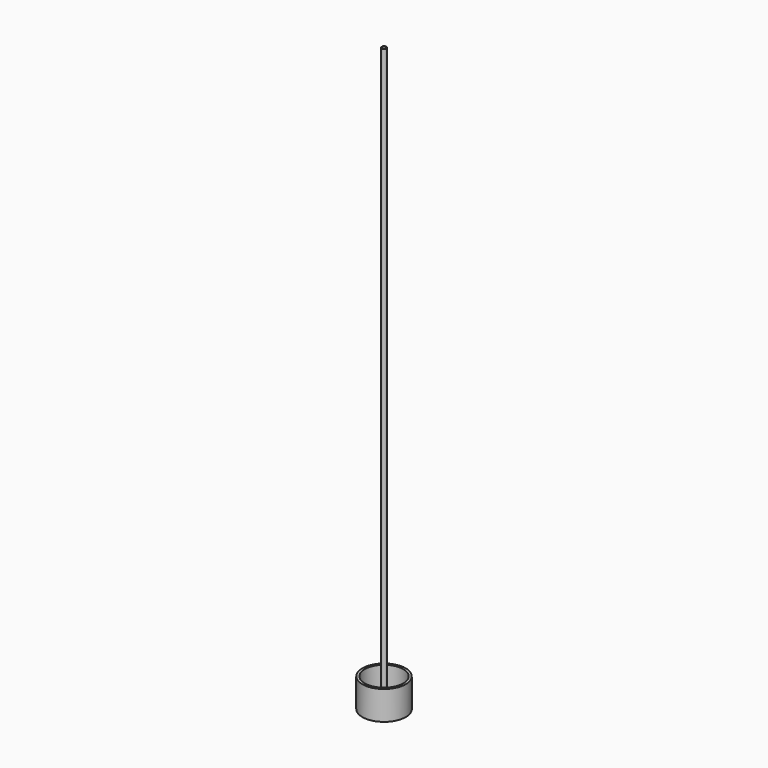
from build123d import *

# Parameters (mm, degrees)
F0_R     = 57.15
F1_DEPTH = 76.2
F2_R     = 50.8
F3_DEPTH = 63.5
F4_R     = 6.35
F4_R_2   = 5.08
F5_DEPTH = 1524


# Not quite as in the source:
# - a fillet or chamfer that OpenCascade refuses, or shapes differently, is made with other operations: its cross-section is extruded or revolved along the edge and cut away or added


with BuildPart() as f1:
    # F0 (on Top) → F1 (new body)
    with BuildSketch(Plane.XY):
        Circle(F0_R)
    extrude(amount=F1_DEPTH)

    # F2 (on face) → F3 (cut)
    with BuildSketch(Plane.XY.offset(76.2)):
        Circle(F2_R)
    extrude(amount=-F3_DEPTH, mode=Mode.SUBTRACT)

    # F4 (on face) → F5 (join)
    with BuildSketch(Plane.XY.offset(12.7)):
        Circle(F4_R)
        Circle(F4_R_2, mode=Mode.SUBTRACT)
    extrude(amount=F5_DEPTH)

    # F6: chamfer of 2.54 on 1 edges, made by hand

    # F6_s1 → F6_t2 (revolve, cut)
    with BuildSketch(Plane.XZ):
        Polygon((6.35, 1534.16), (3.81, 1536.7), (6.35, 1536.7), align=None)
    revolve(axis=Axis((0, 0, 1536.7), (0, 0, 1)), mode=Mode.SUBTRACT)


solid = f1.part
